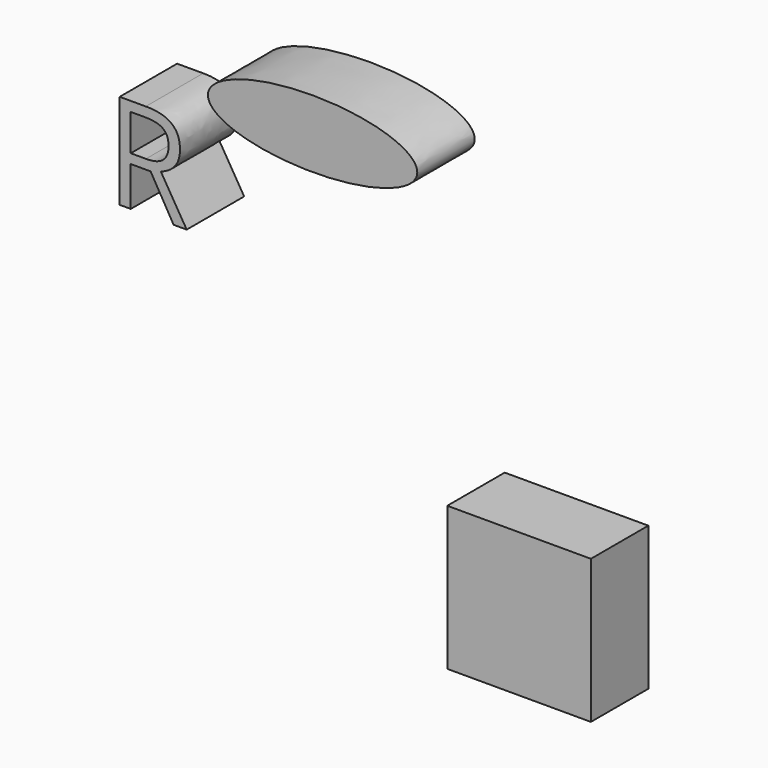
from build123d import *

# Parameters (mm, degrees)
F0_W         = 50
F0_H         = 50
F1_DEPTH     = 25
F2_TEXT_SIZE = 46.3988373263
F3_DEPTH     = 25
F5_DEPTH     = 25


# Not quite as in the source:
# - Text() gives the source's letters only with a copy of the font that has no kerning and outlines rounded to 1/6400 em; it was checked with that copy


with BuildPart() as f1:
    # F0 (on Front) → F1 (new body)
    with BuildSketch(Plane.XZ):
        with Locations((4.0394254029, -39.7594682872)):
            Rectangle(F0_W, F0_H)
    extrude(amount=F1_DEPTH)


with BuildPart() as f3:
    # F2 (on Front) → F3 (new body)
    with BuildSketch(Plane.XZ):
        with Locations((-139.5761370659, 40.3669886291)):
            Text('R', F2_TEXT_SIZE, font='Open Sans', text_align=(TextAlign.LEFT, TextAlign.BOTTOM))
    extrude(amount=F3_DEPTH)


with BuildPart() as f5:
    # F4 (on Front) → F5 (new body)
    with BuildSketch(Plane.XZ):
        with BuildLine():
            add(Edge.make_bspline(
                [(-31.4105860889, 84.0268954635), (-31.4105860889, 104.432002606), (-86.0768500715, 94.2294490347), (-140.7431140542, 84.0268954635), (-86.0768500715, 73.8243418922), (-31.4105860889, 63.621788321), (-31.4105860889, 84.0268954635)],
                knots=[0, 0, 0, 2.0943951024, 2.0943951024, 4.1887902048, 4.1887902048, 6.2831853072, 6.2831853072, 6.2831853072], degree=2, weights=[1, 0.5, 1, 0.5, 1, 0.5, 1]))
        make_face()
    extrude(amount=F5_DEPTH)


solid = Compound([f1.part, f3.part, f5.part])
